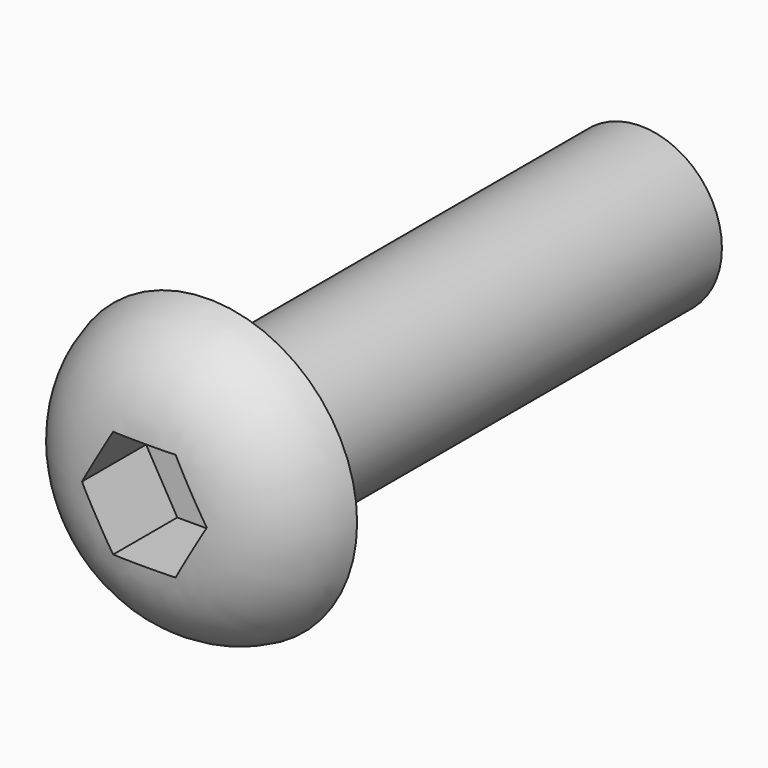
from build123d import *

# Parameters (mm, degrees)
F0_R     = 1.5
F1_DEPTH = 10
F2_R     = 2.75
F3_DEPTH = 1.5
F5_DEPTH = 1.5


# Not quite as in the source:
# - a fillet or chamfer that OpenCascade refuses, or shapes differently, is made with other operations: its cross-section is extruded or revolved along the edge and cut away or added


with BuildPart() as f1:
    # F0 (on Front) → F1 (new body)
    with BuildSketch(Plane.XZ):
        Circle(F0_R)
    extrude(amount=F1_DEPTH)

    # F2 (on face) → F3 (join)
    with BuildSketch(Plane.XZ.offset(10)):
        Circle(F2_R)
    extrude(amount=F3_DEPTH)

    # F4 (on face) → F5 (cut)
    with BuildSketch(Plane.XZ.offset(11.5)):
        Polygon((-0.5773502692, -1), (0.5773502692, -1), (1.1547005384, 0), (0.5773502692, 1), (-0.5773502692, 1), (-1.1547005384, 0), align=None)
    extrude(amount=-F5_DEPTH, mode=Mode.SUBTRACT)

    # F6: fillet of radius 1.9 on 1 edges, made by hand

    # F6_s1 → F6_t2 (revolve, cut)
    with BuildSketch(Plane.XY):
        with BuildLine():
            ThreePointArc((2.75, -10), (2.0863160765, -11.0781745499), (0.8925824379, -11.5))
            Line((0.8925824379, -11.5), (2.75, -11.5))
            Line((2.75, -11.5), (2.75, -10))
        make_face()
    revolve(axis=Axis((0, -11.5, 0), (0, -1, 0)), mode=Mode.SUBTRACT)


solid = f1.part
